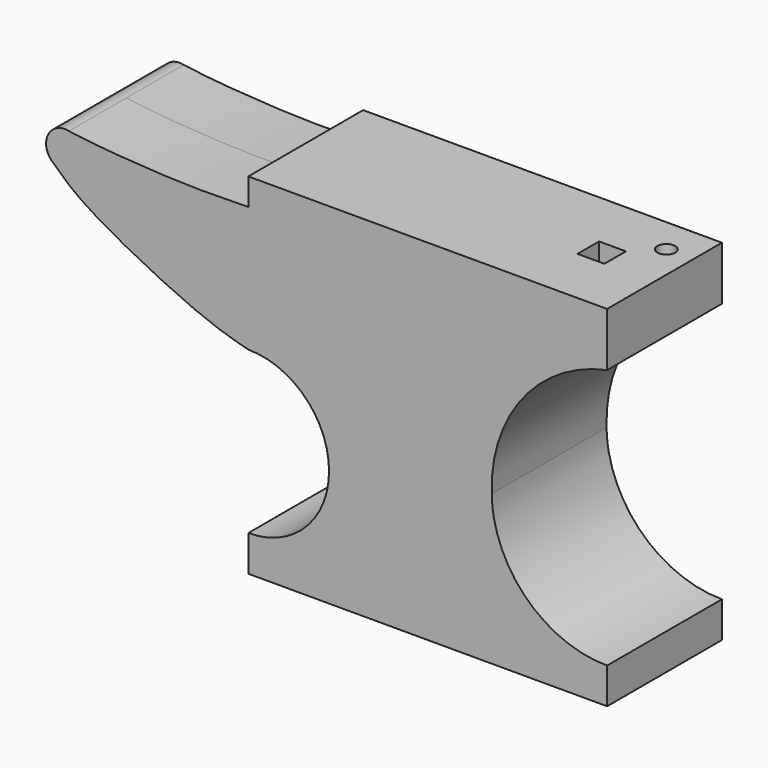
from build123d import *

# Parameters (mm, degrees)
F0_W     = 254
F0_H     = 19.05
F1_DEPTH = 50.8
F2_DEPTH = 50.8
F4_W     = 19.05
F4_H     = 19.05
F4_R     = 6.35
F5_DEPTH = 127
F7_DEPTH = 50.8


# Not quite as in the source:
# - a feature names something its author has since deleted; it is built from what else it names


with BuildPart() as f1:
    # F0 (on Front) → F1 (new body)
    with BuildSketch(Plane.XZ):
        with Locations((0, 111.1250000177)):
            Rectangle(F0_W, F0_H)
    extrude(amount=F1_DEPTH)

    # F0 (on Front) → F2 (join, through all)
    with BuildSketch(Plane.XZ):
        with BuildLine():
            Line((127, 82.5500000177), (127, 101.6000000177))
            Line((127, 101.6000000177), (-127, 101.6000000177))
            Line((-127, 101.6000000177), (-127, 12.7000000177))
            ThreePointArc((-127, 12.7000000177), (-69.8499999823, -44.45), (-127, -101.6000000177))
            Line((-127, -101.6000000177), (-127, -127.0000000177))
            Line((-127, -127.0000000177), (-101.6, -127.0000000177))
            Line((-101.6, -127.0000000177), (88.9, -127.0000000177))
            Line((88.9, -127.0000000177), (127, -127.0000000177))
            Line((127, -127.0000000177), (127, -101.6000000177))
            ThreePointArc((127, -101.6000000177), (75.1661658016, -83.0433945651), (46.8866745136, -35.8060751437))
            ThreePointArc((46.8866745136, -35.8060751437), (45.7784438509, -28.4901624232), (45.3368966297, -21.1039732713))
            ThreePointArc((45.3368966297, -21.1039732713), (67.248156143, 45.6292415321), (127, 82.5500000177))
        make_face()
    extrude(amount=F2_DEPTH)

    # F3: F1 across face


with BuildPart() as f1_1:
    add(f1.part)
    add(f1.part.mirror(Plane(origin=(-11.712184673, 0, 3.7973817679), x_dir=(1, 0, 0), z_dir=(0, 1, 0))))

    # F4 (on Top) → F5 (cut)
    with BuildSketch(Plane.XY):
        with Locations((82.55, 0)):
            Rectangle(F4_W, F4_H)
        with Locations((107.95, 25.4)):
            Circle(F4_R)
    extrude(amount=F5_DEPTH, mode=Mode.SUBTRACT)



with BuildPart() as f7:
    # F0 (on Front) → F7 (new body)
    with BuildSketch(Plane.XZ):
        with BuildLine():
            Line((-127, 12.7000000177), (-127, 101.6000000177))
            add(Edge.make_bspline(
                [(-127, 101.6000000177), (-143.1548670141, 101.1279175586), (-178.3487321582, 100.5000750149), (-235.9685551739, 104.8555928403), (-254, 107.5927615166)],
                knots=[0, 0, 0, 0, 0.4585605976, 1, 1, 1, 1], degree=3))
            ThreePointArc((-254, 107.5927615166), (-268.9111687536, 100.3097468732), (-265.0851011276, 84.1621011496))
            add(Edge.make_bspline(
                [(-265.0851011276, 84.1621011496), (-258.982913814, 78.2797981737), (-242.4670319791, 62.3590460812), (-161.6065585576, 21.8898515634), (-136.6674442933, 15.2672145631), (-127, 12.7000000177)],
                knots=[0, 0, 0, 0, 0.2640715847, 0.7147231864, 1, 1, 1, 1], degree=3))
        make_face()
    extrude(amount=F7_DEPTH)


with BuildPart() as f1_2:
    add(f1_1.part)

    add(f7.part)  # F6 merges F7
    # F6: F7 across plane
    add(f7.part.mirror(Plane.XZ))


solid = f1_2.part
